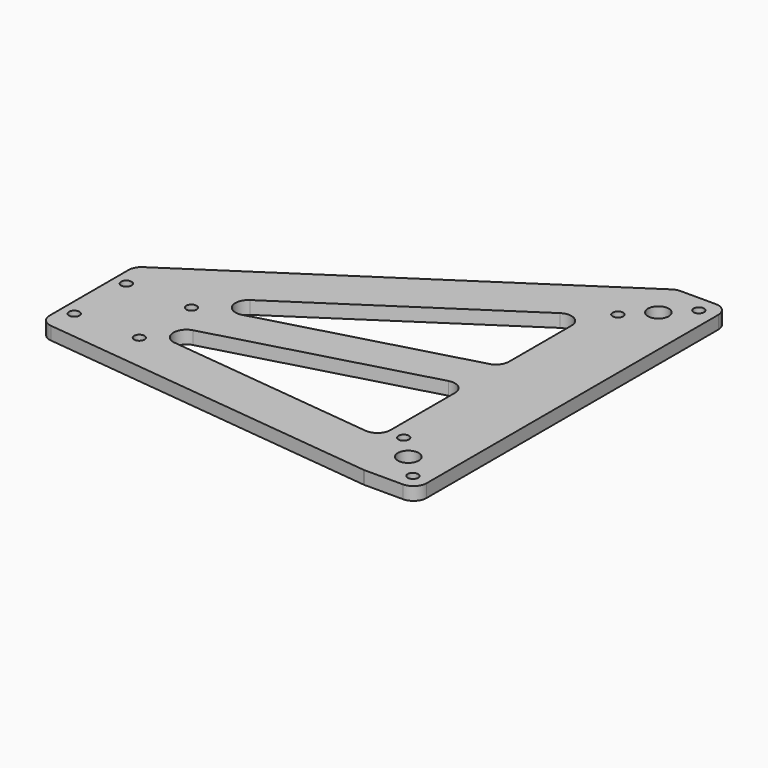
from build123d import *

# Parameters (mm, degrees)
F1_DEPTH = 6.35
F2_R     = 6.35
F3_D     = 10.16
F4_D     = 5.08


with BuildPart() as f1:
    # F0 (on Top) → F1 (new body)
    with BuildSketch(Plane.XY):
        Polygon((99.21875, -63.5), (99.21875, 127), (73.81875, 127), (-99.21875, 12.7), (-99.21875, -15.2791400352), (-99.21875, -20.9632049465), (-99.21875, -44.45), (73.81875, -63.5), align=None)
        Polygon((61.11875, -38.6150398089), (-80.955676291, -22.9738185659), (61.11875, 16.1292345417), align=None, mode=Mode.SUBTRACT)
        Polygon((61.11875, 35.8875947884), (-80.955676291, -3.2154583192), (61.11875, 90.6318691391), align=None, mode=Mode.SUBTRACT)
    extrude(amount=F1_DEPTH)

    # F2
    f2_edges = [f1.edges().sort_by_distance(p)[0] for p in [
        (99.21875, -63.5, 3.175),
        (99.21875, 127, 3.175),
        (-80.955676, -3.215458, 3.175),
        (-80.955676, -22.973819, 3.175),
        (61.11875, 90.631869, 3.175),
        (61.11875, 16.129235, 3.175),
        (61.11875, -38.61504, 3.175),
        (61.11875, 35.887595, 3.175),
        (-99.21875, -44.45, 3.175),
        (73.81875, -63.5, 3.175),
        (73.81875, 127, 3.175),
        (-99.21875, 12.7, 3.175),
    ]]
    fillet(f2_edges, radius=F2_R)

    # F3 (through all)
    with Locations(Plane(origin=(0, 0, 0), x_dir=(1, 0, 0), z_dir=(0, 0, -1))):
        with Locations((80.16875, -107.95), (80.16875, 44.45)):
            Hole(F3_D / 2)

    # F4 (through all)
    with Locations(Plane(origin=(0, 0, 0), x_dir=(1, 0, 0), z_dir=(0, 0, -1))):
        with Locations((91.1368808609, -118.9181308609), (69.2006191391, -96.9818691391), (91.3940701513, 55.6753201513), (68.9434298487, 33.2246798487), (-61.11875, 31.75), (-92.86875, 0), (-61.11875, 0), (-92.86875, 31.75)):
            Hole(F4_D / 2)


solid = f1.part
